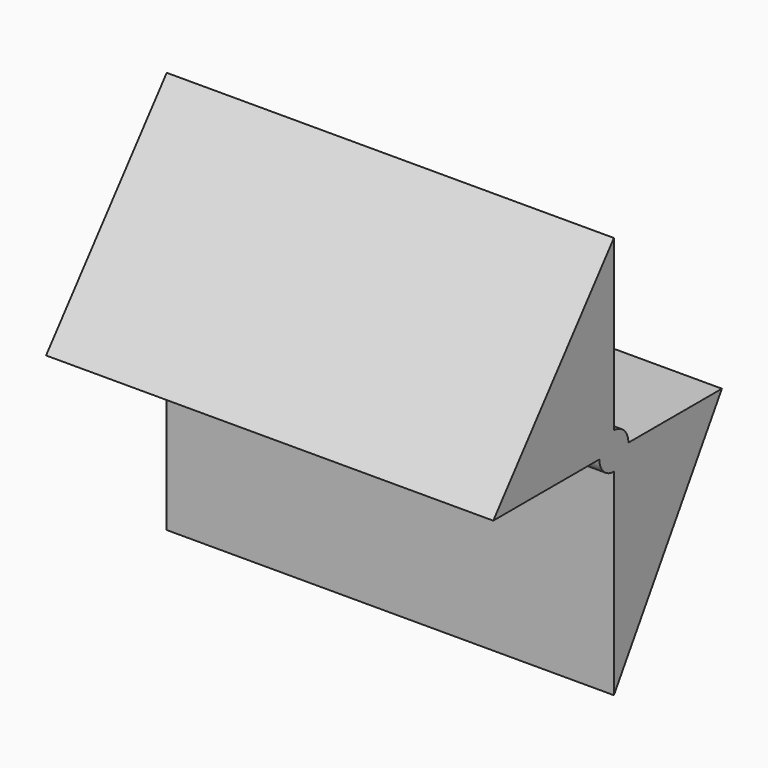
from build123d import *

# Parameters (mm, degrees)
F2_DEPTH      = 115.1771843433
F2_DEPTH_BACK = 52.7988504618


# Not quite as in the source:
# - the program builds the solid bodies; features that only make, move or delete a surface that nothing else refers to are left out


with BuildPart() as f2:
    # F0 (on Right) → F2 (new body, two sides)
    with BuildSketch(Plane.YZ) as f2_sk:
        with BuildLine():
            Line((0, 70.4632103443), (-56.6462948918, 0))
            Line((-56.6462948918, 0), (-6.8218263729, 0))
            ThreePointArc((-6.8218263729, 0), (-4.8237596884, -4.8237596884), (0, -6.8218263729))
            Line((0, -6.8218263729), (0, -80.7569846511))
            Line((0, -80.7569846511), (50.7276728749, 0))
            Line((50.7276728749, 0), (6.8218263729, 0))
            ThreePointArc((6.8218263729, 0), (4.8237596884, 4.8237596884), (0, 6.8218263729))
            Line((0, 6.8218263729), (0, 16.5492296219))
            Line((0, 16.5492296219), (0, 70.4632103443))
        make_face()
    extrude(amount=F2_DEPTH)
    extrude(f2_sk.sketch, amount=-F2_DEPTH_BACK)


solid = f2.part
